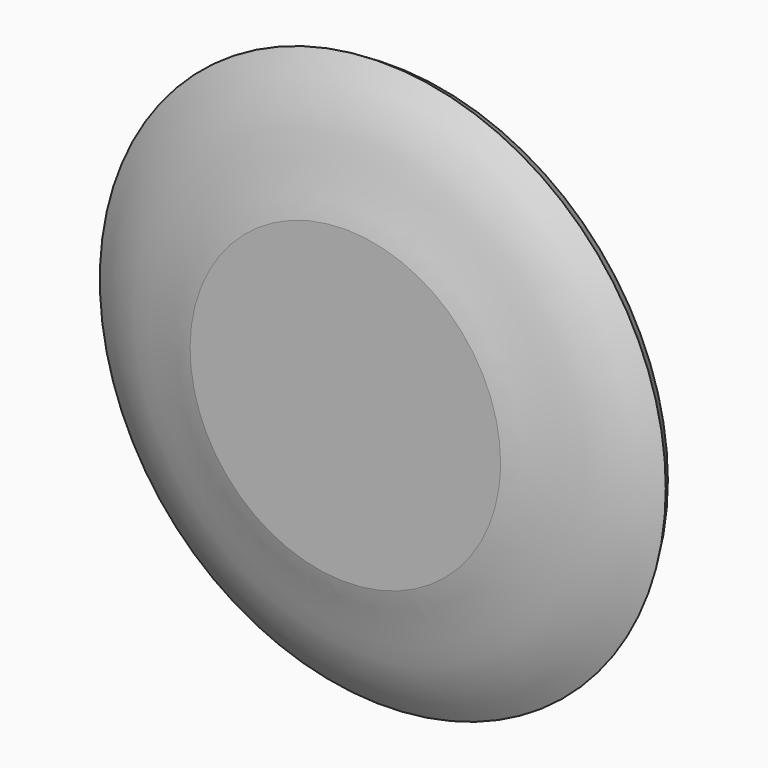
from build123d import *

# Parameters (mm, degrees)
F3_DEPTH = 1.27


# Not quite as in the source:
# - the dataset's text gives a spline's control points without its knots; the knots are read off the source's solid


with BuildPart() as f1:
    # F0 (on Top) → F1 (revolve)
    with BuildSketch(Plane.XY):
        with BuildLine():
            Line((0, 3.175), (0, 0))
            Line((0, 0), (0.0483732221, 0.126777769))
            add(Edge.make_bspline(
                [(0.0483732221, 0.1267777671), (2.1425433468, 0.1181949129), (6.4413258481, 0.0890337964), (12.9108112798, 0.0620545487), (19.1525366078, 0.1064268527), (23.9368157495, 0.2489309341), (27.3993505655, 0.4567479093), (29.7877305037, 0.6675796116), (31.9566435279, 0.9485179212), (33.8570376049, 1.2999888181), (35.5368416593, 1.69897799), (37.0371573939, 2.1219862961), (38.4015343875, 2.5419205888), (39.4751540886, 2.8731693163), (40.3256085154, 3.119672766), (40.9906733706, 3.3016750857), (41.6830106743, 3.4830815946), (42.6350739841, 3.724489538), (43.8698571739, 4.027813647), (45.3922972671, 4.4027417127), (46.6722427938, 4.7329949415), (47.689990497, 5.0138614605), (48.4490127923, 5.2351298254), (49.1948201109, 5.4671266007), (50.1646945957, 5.7882307085), (51.337715765, 6.212770994), (52.690143853, 6.758306314), (54.4315564533, 7.5320961824), (56.5186693938, 8.5846645619), (58.9364068625, 9.9592448244), (60.5161655926, 10.9272420375), (61.3055767878, 11.419646447)],
                knots=[0.0005982269, 0.0005982269, 0.0005982269, 0.0005982269, 0.0625, 0.125, 0.1875, 0.25, 0.28125, 0.3125, 0.34375, 0.375, 0.40625, 0.4375, 0.46875, 0.5, 0.515625, 0.53125, 0.546875, 0.5625, 0.59375, 0.625, 0.65625, 0.671875, 0.6875, 0.703125, 0.71875, 0.75, 0.78125, 0.8125, 0.875, 0.9375, 0.9999998063, 0.9999998063, 0.9999998063, 0.9999998063], degree=3))
            Line((61.3055767878, 11.419646447), (59.6924508727, 14.0057881257))
            add(Edge.make_bspline(
                [(0, 3.175), (11.3313598558, 3.1291642226), (30.5330430918, 2.7907248238), (38.8639839953, 6.1128612906), (47.6584070453, 7.9242497832), (53.9757361198, 10.5463281379), (57.7714374215, 12.8075335236), (59.6924508727, 14.0057881257)],
                knots=[0, 0, 0, 0, 0.3341820731, 0.5122398896, 0.6874928788, 0.8452121481, 1, 1, 1, 1], degree=3))
        make_face()
    revolve(axis=Axis((0, 1.5875, 0), (0, 1, 0)))

    # F2 (on Front) → F3 (cut, symmetric)
    with BuildSketch(Plane.XZ):
        Polygon((-63.8710334897, -66.6622146964), (-51.9457645714, -66.154755652), (56.3966184855, -66.154755652), (56.3966184855, 62.9934221506), (-63.8710334897, 62.9934221506), align=None)
    extrude(amount=F3_DEPTH, both=True, mode=Mode.SUBTRACT)


solid = f1.part
